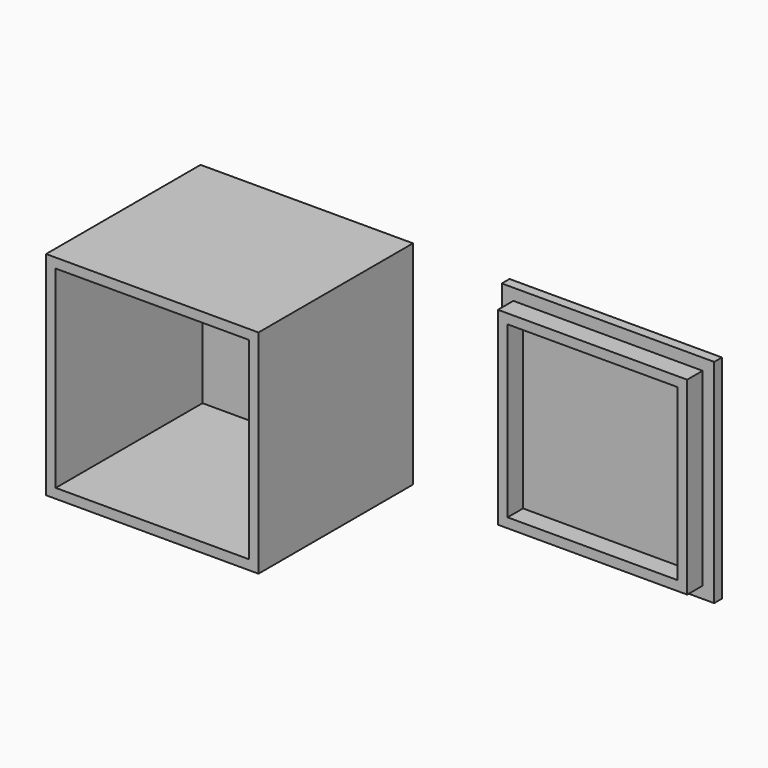
from build123d import *

# Parameters (mm, degrees)
F0_W     = 22
F0_H     = 22
F0_W_2   = 20
F0_H_2   = 20
F1_DEPTH = 1
F0_W_3   = 19.6
F0_H_3   = 19.6
F0_W_4   = 17.6
F0_H_4   = 17.6
F2_DEPTH = 20
F3_DEPTH = 3


with BuildPart() as f1:
    # F0 (on Front) → F1 (new body)
    with BuildSketch(Plane.XZ):
        with Locations((11, 11)):
            Rectangle(F0_W, F0_H)
        with Locations((11, 11)):
            Rectangle(F0_W_2, F0_H_2, mode=Mode.SUBTRACT)
        with Locations((11, 11)):
            Rectangle(F0_W_2, F0_H_2)
    extrude(amount=F1_DEPTH)

    # F0 (on Front) → F2 (join)
    with BuildSketch(Plane.XZ):
        with Locations((11, 11)):
            Rectangle(F0_W, F0_H)
        with Locations((11, 11)):
            Rectangle(F0_W_2, F0_H_2, mode=Mode.SUBTRACT)
    extrude(amount=F2_DEPTH)


with BuildPart() as f1b:
    # F0 (on Front) → F1, piece 2 (new body)
    with BuildSketch(Plane.XZ):
        with Locations((43, 11)):
            Rectangle(F0_W, F0_H)
        with Locations((43, 11)):
            Rectangle(F0_W_3, F0_H_3, mode=Mode.SUBTRACT)
        with Locations((43, 11)):
            Rectangle(F0_W_3, F0_H_3)
        with Locations((43, 11)):
            Rectangle(F0_W_4, F0_H_4, mode=Mode.SUBTRACT)
        with Locations((43, 11)):
            Rectangle(F0_W_4, F0_H_4)
    extrude(amount=F1_DEPTH)

    # F0 (on Front) → F3 (join)
    with BuildSketch(Plane.XZ):
        with Locations((43, 11)):
            Rectangle(F0_W_3, F0_H_3)
        with Locations((43, 11)):
            Rectangle(F0_W_4, F0_H_4, mode=Mode.SUBTRACT)
    extrude(amount=F3_DEPTH)


solid = Compound([f1.part, f1b.part])
